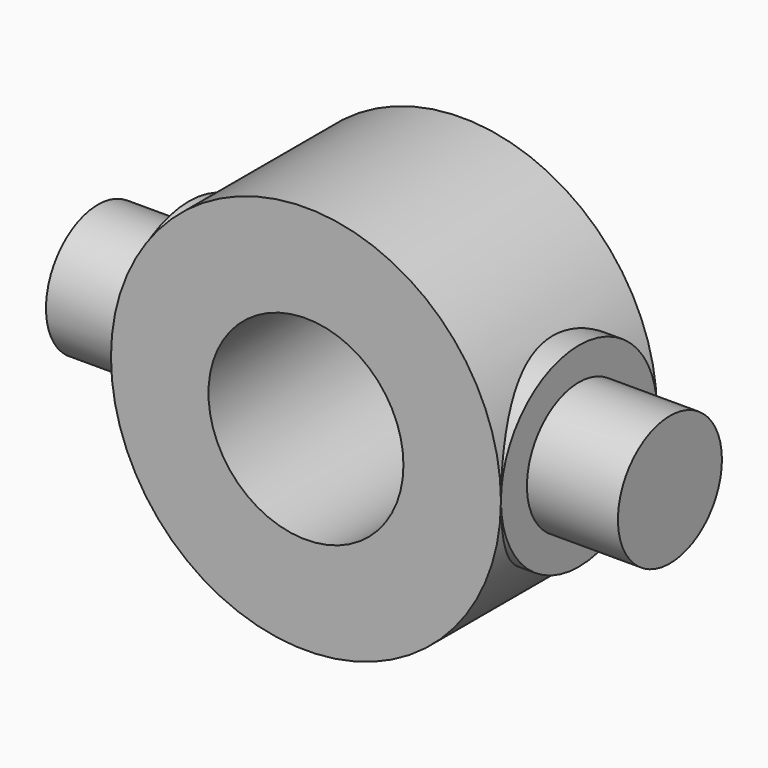
from build123d import *

# Parameters (mm, degrees)
F0_R     = 15
F1_DEPTH = 7.5
F2_R     = 7.5
F3_DEPTH = 15
F4_R     = 5
F5_DEPTH = 22
F6_R     = 7.5
F7_DEPTH = 15.0010001


with BuildPart() as f1:
    # F0 (on Front) → F1 (new body, symmetric)
    with BuildSketch(Plane.XZ):
        Circle(F0_R)
    extrude(amount=F1_DEPTH, both=True)

    # F2 (on Right) → F3 (join, symmetric)
    with BuildSketch(Plane.YZ):
        Circle(F2_R)
    extrude(amount=F3_DEPTH, both=True)

    # F4 (on Right) → F5 (join, symmetric)
    with BuildSketch(Plane.YZ):
        Circle(F4_R)
    extrude(amount=F5_DEPTH, both=True)

    # F6 (on face) → F7 (cut, through all)
    with BuildSketch(Plane.XZ.offset(7.5)):
        Circle(F6_R)
    extrude(amount=-F7_DEPTH, mode=Mode.SUBTRACT)


solid = f1.part
